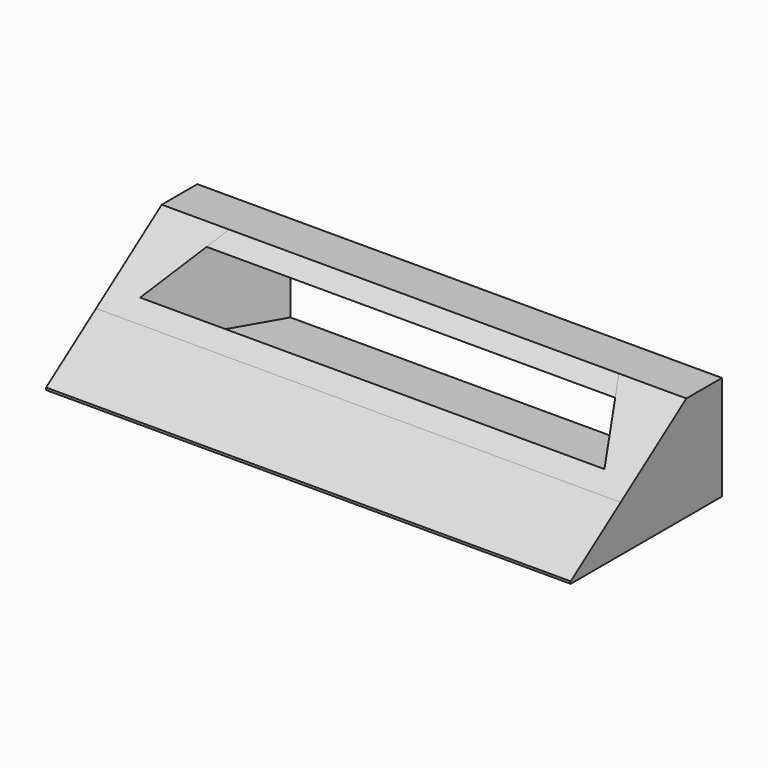
from build123d import *

# Parameters (mm, degrees)
F1_DEPTH    = 30
F2_T1_DEPTH = 326.8852689227
F3_DEPTH    = 30
F0_W        = 180.7846096908
F0_H        = 21.5329241753
F6_DEPTH    = 25
F7_DEPTH    = 6
F5_W        = 259.5228254795
F5_H        = 121.416632086
F8_DEPTH    = 25
F9_DEPTH    = 26


# Not quite as in the source:
# - a fillet or chamfer that OpenCascade refuses, or shapes differently, is made with other operations: its cross-section is extruded or revolved along the edge and cut away or added


with BuildPart() as f1:
    # F0 (on Top) → F1 (new body)
    with BuildSketch(Plane.XY):
        Polygon((80, -24), (-80, -24), (-58.2867488807, 13.6084541361), (-65.214952111, 13.6084541361), (-73.0717967697, 0), (-90.3923048454, -30), (90.3923048454, -30), (73.0717967697, 0), (65.214952111, 13.6084541361), (58.2867488807, 13.6084541361), align=None)
        Polygon((-90.3923048454, -30), (-73.0717967697, 0), (-90.3923048454, 0), align=None)
        Polygon((90.3923048454, 0), (73.0717967697, 0), (90.3923048454, -30), align=None)
        Polygon((-73.0717967697, 0), (-65.214952111, 13.6084541361), (-90.3923048454, 13.6084541361), (-90.3923048454, 0), align=None)
        Polygon((90.3923048454, 13.6084541361), (65.214952111, 13.6084541361), (73.0717967697, 0), (90.3923048454, 0), align=None)
    extrude(amount=F1_DEPTH)

    # F2: chamfer of 20 x 28.2888686106 on 1 edges, made by hand

    # F2_s2 → F2_t1 (cut)
    with BuildSketch(Plane.YZ.offset(-163.4426344613)):
        Polygon((-30, 10), (-1.7111313894, 30), (-30, 30), align=None)
    extrude(amount=F2_T1_DEPTH, mode=Mode.SUBTRACT)

    # F0 (on Top) → F3 (join)
    with BuildSketch(Plane.XY):
        Polygon((-58.2867488807, 13.6084541361), (-80, -24), (80, -24), (58.2867488807, 13.6084541361), align=None)
    extrude(amount=F3_DEPTH)

    # F0 (on Top) → F6 (join)
    with BuildSketch(Plane.XY):
        with Locations((0, -40.7664620876)):
            Rectangle(F0_W, F0_H)
    extrude(amount=F6_DEPTH)

    # F0 (on Top) → F7 (join)
    with BuildSketch(Plane.XY):
        Polygon((-58.2867488807, 13.6084541361), (-80, -24), (80, -24), (58.2867488807, 13.6084541361), align=None)
        Polygon((80, -24), (-80, -24), (-58.2867488807, 13.6084541361), (-65.214952111, 13.6084541361), (-73.0717967697, 0), (-90.3923048454, -30), (90.3923048454, -30), (73.0717967697, 0), (65.214952111, 13.6084541361), (58.2867488807, 13.6084541361), align=None)
        Polygon((-90.3923048454, -30), (-73.0717967697, 0), (-90.3923048454, 0), align=None)
        Polygon((-73.0717967697, 0), (-65.214952111, 13.6084541361), (-90.3923048454, 13.6084541361), (-90.3923048454, 0), align=None)
        Polygon((90.3923048454, 13.6084541361), (65.214952111, 13.6084541361), (73.0717967697, 0), (90.3923048454, 0), align=None)
        Polygon((90.3923048454, 0), (73.0717967697, 0), (90.3923048454, -30), align=None)
        with Locations((0, -40.7664620876)):
            Rectangle(F0_W, F0_H)
    extrude(amount=-F7_DEPTH)

    # F5 (on offset) → F8 (cut)
    with BuildSketch(Plane(origin=(0, -14.7116228469, 20.8087582883), x_dir=(1, 0, 0), z_dir=(0, -0.5772877121, 0.8165408119))):
        with Locations((5.841344595, -0.7894355804)):
            Rectangle(F5_W, F5_H)
    extrude(amount=F8_DEPTH, mode=Mode.SUBTRACT)

    # F0 (on Top) → F9 (cut)
    with BuildSketch(Plane.XY):
        Polygon((-58.2867488807, 13.6084541361), (-80, -24), (80, -24), (58.2867488807, 13.6084541361), align=None)
    extrude(amount=F9_DEPTH, mode=Mode.SUBTRACT)


solid = f1.part
